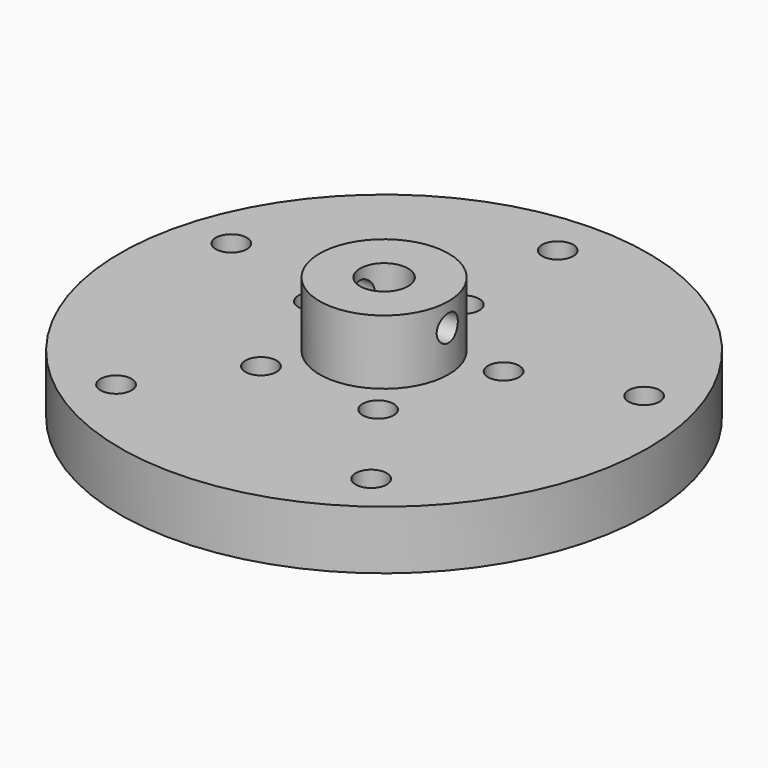
from build123d import *

# Parameters (mm, degrees)
F0_R     = 45
F1_DEPTH = 10
F2_R     = 11
F3_DEPTH = 11
F5_D     = 8.2
F7_D     = 5.3
F8_R     = 2.25
F9_DEPTH = 50


# Not quite as in the source:
# - a feature names something its author has since deleted; it is built from what else it names


with BuildPart() as f1:
    # F0 (on Top) → F1 (new body)
    with BuildSketch(Plane.XY):
        Circle(F0_R)
    extrude(amount=F1_DEPTH)

    # F2 (on face) → F3 (join)
    with BuildSketch(Plane.XY.offset(10)):
        Circle(F2_R)
    extrude(amount=F3_DEPTH)

    # F5 (through all)
    with Locations(Plane.XY.offset(21)):
        with Locations((0, 0)):
            Hole(F5_D / 2)

    # F7 (through all)
    with Locations(Plane.XY.offset(10)):
        with Locations((0, 17), (16.167960777, 5.2532889044), (9.992349289, -13.7532889044), (-9.992349289, -13.7532889044), (-16.167960777, 5.2532889044), (35.1890911029, 11.4336287919), (21.7480543348, -29.9336287919), (-21.7480543348, -29.9336287919), (-35.1890911029, 11.4336287919), (0, 37)):
            Hole(F7_D / 2)

    # F8 (on Right) → F9 (cut, symmetric)
    with BuildSketch(Plane.YZ):
        with Locations((0, 17)):
            Circle(F8_R)
    extrude(amount=F9_DEPTH, both=True, mode=Mode.SUBTRACT)


solid = f1.part
